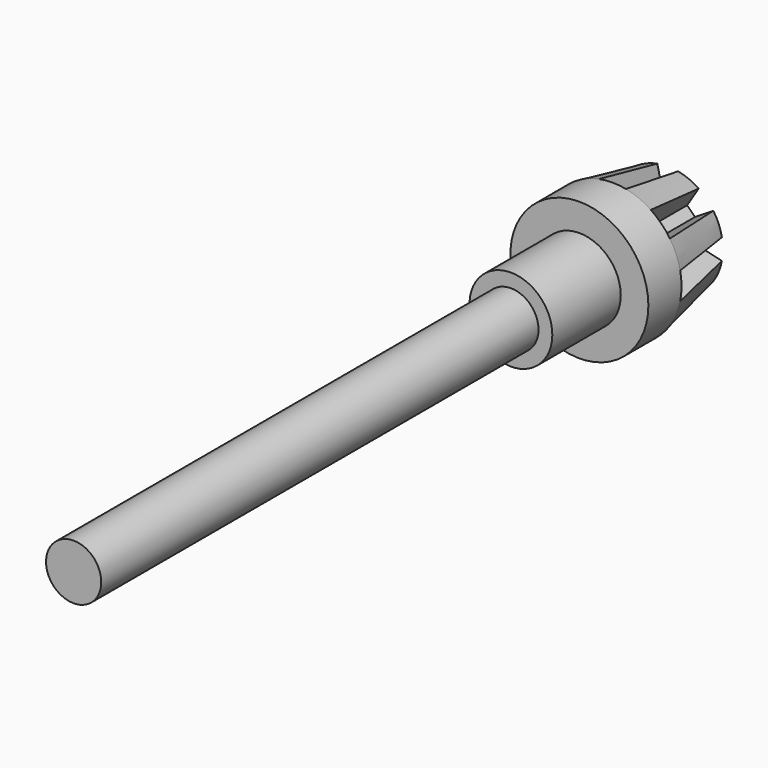
from build123d import *

# Parameters (mm, degrees)
F0_R            = 25
F1_DEPTH        = 40
F2_SIZE2        = 5
F2_SIZE         = 25
F7_COPIES_COUNT = 8
F8_R            = 15
F9_DEPTH        = 31
F10_R           = 10
F11_DEPTH       = 198


# Not quite as in the source:
# - a pattern or mirror of a feature is missing from the dataset's text; its kind, count and spacing are read off the source's solid


with BuildPart() as f1:
    # F0 (on Front) → F1 (new body)
    with BuildSketch(Plane.XZ):
        Circle(F0_R)
    extrude(amount=F1_DEPTH)

    # F2
    f2_edges = [f1.edges().sort_by_distance(p)[0] for p in [
        (-25, 0, 0),
    ]]
    f2_side = f1.faces().sort_by_distance((-25, -20, 0))[0]
    chamfer(f2_edges, length=F2_SIZE, length2=F2_SIZE2, reference=f2_side)

    # F4 (on Front) → F7 section 0
    with BuildSketch(Plane.XZ):
        Polygon((8, -38), (2, -12), (-2, -12), (-8, -38), align=None)
    # F5 (on offset) → F7 section 1
    with BuildSketch(Plane.XZ.offset(25)):
        Polygon((8, -38), (2, -12), (-2, -12), (-8, -38), align=None)
    f7 = loft(mode=Mode.SUBTRACT)

    # F7_copies: F7 ×8 about axis
    f7_copies_axis = Axis((0, 0, 0), (0, 1, 0))
    for i in range(1, F7_COPIES_COUNT):
        add(f7.rotate(f7_copies_axis, i * 360 / F7_COPIES_COUNT), mode=Mode.SUBTRACT)

    # F8 (on face) → F9 (join)
    with BuildSketch(Plane.XZ.offset(40)):
        Circle(F8_R)
    extrude(amount=F9_DEPTH)

    # F10 (on face) → F11 (join)
    with BuildSketch(Plane.XZ.offset(71)):
        Circle(F10_R)
    extrude(amount=F11_DEPTH)


solid = f1.part
